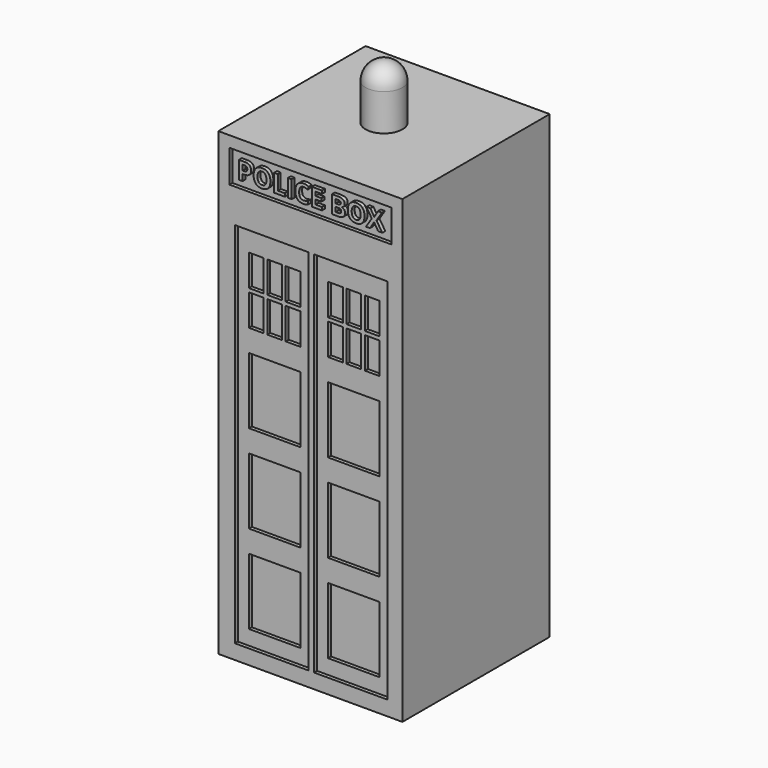
from build123d import *

# Parameters (mm, degrees)
F0_W      = 50
F0_H      = 50
F1_DEPTH  = 125
F6_W      = 44
F6_H      = 8.8186975504
F6_W_2    = 1.0133068417
F6_H_2    = 4.7779143029
F7_DEPTH  = 1
F6_W_3    = 4
F6_H_3    = 8.5
F6_W_4    = 14
F6_H_4    = 18
F8_DEPTH  = 2
F6_W_5    = 20
F6_H_5    = 100
F9_DEPTH  = 1
F11_W     = 44
F11_H     = 22
F11_W_2   = 1.2572977775
F11_H_2   = 4.6096520825
F11_H_3   = 6.4157807891
F12_DEPTH = 1


with BuildPart() as f1:
    # F0 (on Top) → F1 (new body)
    with BuildSketch(Plane.XY):
        Rectangle(F0_W, F0_H)
    extrude(amount=F1_DEPTH)

    # F3 (on Front) → F4 (revolve)
    with BuildSketch(Plane.XZ):
        with BuildLine():
            Line((0, 125), (0, 140))
            ThreePointArc((0, 140), (-3.5355339059, 138.5355339059), (-5, 135))
            Line((-5, 135), (-5, 125))
            Line((-5, 125), (0, 125))
        make_face()
    revolve(axis=Axis((0, 0, 66.3798125461), (0, 0, 1)))

    # F6 (on offset) → F7 (cut)
    with BuildSketch(Plane.XZ.offset(25)):
        with Locations((0, 117.5906512248)):
            Rectangle(F6_W, F6_H)
        with BuildLine():
            add(Edge.make_bspline(
                [(-16.5506784136, 119.584847455), (-16.0984026561, 119.2104781574), (-16.0984026561, 118.4690596324)],
                knots=[0, 0, 0, 1, 1, 1], degree=2))
            add(Edge.make_bspline(
                [(-16.0984026561, 118.4690596324), (-16.0984026561, 117.6973151029), (-16.580481556, 117.2889597658)],
                knots=[0, 0, 0, 1, 1, 1], degree=2))
            add(Edge.make_bspline(
                [(-16.580481556, 117.2889597658), (-17.0625604559, 116.8806044286), (-17.9514261065, 116.8806044286)],
                knots=[0, 0, 0, 1, 1, 1], degree=2))
            Line((-17.9514261065, 116.8806044286), (-18.3854016888, 116.8806044286))
            Line((-18.3854016888, 116.8806044286), (-18.3854016888, 115.1813024496))
            Line((-18.3854016888, 115.1813024496), (-19.3987085305, 115.1813024496))
            Line((-19.3987085305, 115.1813024496), (-19.3987085305, 119.9592167525))
            Line((-19.3987085305, 119.9592167525), (-17.8729967844, 119.9592167525))
            add(Edge.make_bspline(
                [(-17.8729967844, 119.9592167525), (-17.0029541711, 119.9592167525), (-16.5506784136, 119.584847455)],
                knots=[0, 0, 0, 1, 1, 1], degree=2))
        make_face(mode=Mode.SUBTRACT)
        with BuildLine():
            add(Edge.make_bspline(
                [(-11.4428380957, 119.4002771169), (-10.8593239392, 118.7660453321), (-10.8593239392, 117.577056809)],
                knots=[0, 0, 0, 1, 1, 1], degree=2))
            add(Edge.make_bspline(
                [(-10.8593239392, 117.577056809), (-10.8593239392, 116.3901597344), (-11.4475438551, 115.7527907767)],
                knots=[0, 0, 0, 1, 1, 1], degree=2))
            add(Edge.make_bspline(
                [(-11.4475438551, 115.7527907767), (-12.0357637709, 115.115421819), (-13.1337742804, 115.115421819)],
                knots=[0, 0, 0, 1, 1, 1], degree=2))
            add(Edge.make_bspline(
                [(-13.1337742804, 115.115421819), (-14.2317847899, 115.115421819), (-14.8200047058, 115.7527907767)],
                knots=[0, 0, 0, 1, 1, 1], degree=2))
            add(Edge.make_bspline(
                [(-14.8200047058, 115.7527907767), (-15.4082246216, 116.3901597344), (-15.4082246216, 117.5833311547)],
                knots=[0, 0, 0, 1, 1, 1], degree=2))
            add(Edge.make_bspline(
                [(-15.4082246216, 117.5833311547), (-15.4082246216, 118.7765025751), (-14.8184361193, 119.4055057384)],
                knots=[0, 0, 0, 1, 1, 1], degree=2))
            add(Edge.make_bspline(
                [(-14.8184361193, 119.4055057384), (-14.2286476171, 120.0345089017), (-13.1274999346, 120.0345089017)],
                knots=[0, 0, 0, 1, 1, 1], degree=2))
            add(Edge.make_bspline(
                [(-13.1274999346, 120.0345089017), (-12.0263522522, 120.0345089017), (-11.4428380957, 119.4002771169)],
                knots=[0, 0, 0, 1, 1, 1], degree=2))
        make_face(mode=Mode.SUBTRACT)
        Polygon((-6.9179890722, 115.1813024496), (-9.8690230321, 115.1813024496), (-9.8690230321, 119.9592167525), (-8.8557161904, 119.9592167525), (-8.8557161904, 116.0178818854), (-6.9179890722, 116.0178818854), align=None, mode=Mode.SUBTRACT)
        with Locations((-5.5810305613, 117.5702596011)):
            Rectangle(F6_W_2, F6_H_2, mode=Mode.SUBTRACT)
        with BuildLine():
            add(Edge.make_bspline(
                [(-1.3097696792, 119.0896970014), (-1.5806122716, 119.1843350501), (-1.8420433453, 119.1843350501)],
                knots=[0, 0, 0, 1, 1, 1], degree=2))
            add(Edge.make_bspline(
                [(-1.8420433453, 119.1843350501), (-2.4140545345, 119.1843350501), (-2.727771823, 118.7545423649)],
                knots=[0, 0, 0, 1, 1, 1], degree=2))
            add(Edge.make_bspline(
                [(-2.727771823, 118.7545423649), (-3.0414891114, 118.3247496797), (-3.0414891114, 117.5571880474)],
                knots=[0, 0, 0, 1, 1, 1], degree=2))
            add(Edge.make_bspline(
                [(-3.0414891114, 117.5571880474), (-3.0414891114, 115.9593213249), (-1.8420433453, 115.9593213249)],
                knots=[0, 0, 0, 1, 1, 1], degree=2))
            add(Edge.make_bspline(
                [(-1.8420433453, 115.9593213249), (-1.3390499595, 115.9593213249), (-0.6237745418, 116.2102951557)],
                knots=[0, 0, 0, 1, 1, 1], degree=2))
            Line((-0.6237745418, 116.2102951557), (-0.6237745418, 115.3611670283))
            add(Edge.make_bspline(
                [(-0.6237745418, 115.3611670283), (-1.2114715955, 115.115421819), (-1.9372042561, 115.115421819)],
                knots=[0, 0, 0, 1, 1, 1], degree=2))
            add(Edge.make_bspline(
                [(-1.9372042561, 115.115421819), (-2.979791378, 115.115421819), (-3.5319338057, 115.7480850174)],
                knots=[0, 0, 0, 1, 1, 1], degree=2))
            add(Edge.make_bspline(
                [(-3.5319338057, 115.7480850174), (-4.0840762333, 116.3807482157), (-4.0840762333, 117.5634623931)],
                knots=[0, 0, 0, 1, 1, 1], degree=2))
            add(Edge.make_bspline(
                [(-4.0840762333, 117.5634623931), (-4.0840762333, 118.3090638153), (-3.8127107788, 118.8695720373)],
                knots=[0, 0, 0, 1, 1, 1], degree=2))
            add(Edge.make_bspline(
                [(-3.8127107788, 118.8695720373), (-3.5413453243, 119.4300802593), (-3.033123317, 119.7286345455)],
                knots=[0, 0, 0, 1, 1, 1], degree=2))
            add(Edge.make_bspline(
                [(-3.033123317, 119.7286345455), (-2.5249013098, 120.0271888317), (-1.8420433453, 120.0271888317)],
                knots=[0, 0, 0, 1, 1, 1], degree=2))
            add(Edge.make_bspline(
                [(-1.8420433453, 120.0271888317), (-1.1466366892, 120.0271888317), (-0.4439099631, 119.691511333)],
                knots=[0, 0, 0, 1, 1, 1], degree=2))
            Line((-0.4439099631, 119.691511333), (-0.7701759431, 118.8674805887))
            add(Edge.make_bspline(
                [(-0.7701759431, 118.8674805887), (-1.0389270869, 118.9950589527), (-1.3097696792, 119.0896970014)],
                knots=[0, 0, 0, 1, 1, 1], degree=2))
        make_face(mode=Mode.SUBTRACT)
        Polygon((3.1439700923, 116.0178818854), (3.1439700923, 115.1813024496), (0.3926694727, 115.1813024496), (0.3926694727, 119.9592167525), (3.1439700923, 119.9592167525), (3.1439700923, 119.1289116624), (1.4059763143, 119.1289116624), (1.4059763143, 118.0800501948), (3.0237117984, 118.0800501948), (3.0237117984, 117.2497451047), (1.4059763143, 117.2497451047), (1.4059763143, 116.0178818854), align=None, mode=Mode.SUBTRACT)
        with BuildLine():
            Line((5.8795848475, 115.1813024496), (5.8795848475, 119.9592167525))
            Line((5.8795848475, 119.9592167525), (7.3666047946, 119.9592167525))
            add(Edge.make_bspline(
                [(7.3666047946, 119.9592167525), (8.3830488092, 119.9592167525), (8.8421217746, 119.670073985)],
                knots=[0, 0, 0, 1, 1, 1], degree=2))
            add(Edge.make_bspline(
                [(8.8421217746, 119.670073985), (9.30119474, 119.3809312175), (9.30119474, 118.7503594677)],
                knots=[0, 0, 0, 1, 1, 1], degree=2))
            add(Edge.make_bspline(
                [(9.30119474, 118.7503594677), (9.30119474, 118.3216125069), (9.1004156754, 118.0471098795)],
                knots=[0, 0, 0, 1, 1, 1], degree=2))
            add(Edge.make_bspline(
                [(9.1004156754, 118.0471098795), (8.8996366108, 117.7726072521), (8.5660505608, 117.7171838645)],
                knots=[0, 0, 0, 1, 1, 1], degree=2))
            Line((8.5660505608, 117.7171838645), (8.5660505608, 117.6847664113))
            add(Edge.make_bspline(
                [(8.5660505608, 117.6847664113), (9.0198949047, 117.5833311547), (9.2211968315, 117.3056913545)],
                knots=[0, 0, 0, 1, 1, 1], degree=2))
            add(Edge.make_bspline(
                [(9.2211968315, 117.3056913545), (9.4224987582, 117.0280515542), (9.4224987582, 116.5668871402)],
                knots=[0, 0, 0, 1, 1, 1], degree=2))
            add(Edge.make_bspline(
                [(9.4224987582, 116.5668871402), (9.4224987582, 115.913309456), (8.949831377, 115.5473059528)],
                knots=[0, 0, 0, 1, 1, 1], degree=2))
            add(Edge.make_bspline(
                [(8.949831377, 115.5473059528), (8.4771639957, 115.1813024496), (7.6667276673, 115.1813024496)],
                knots=[0, 0, 0, 1, 1, 1], degree=2))
            Line((7.6667276673, 115.1813024496), (5.8795848475, 115.1813024496))
        make_face(mode=Mode.SUBTRACT)
        with BuildLine():
            add(Edge.make_bspline(
                [(14.1293038091, 119.4002771169), (14.7128179655, 118.7660453321), (14.7128179655, 117.577056809)],
                knots=[0, 0, 0, 1, 1, 1], degree=2))
            add(Edge.make_bspline(
                [(14.7128179655, 117.577056809), (14.7128179655, 116.3901597344), (14.1245980497, 115.7527907767)],
                knots=[0, 0, 0, 1, 1, 1], degree=2))
            add(Edge.make_bspline(
                [(14.1245980497, 115.7527907767), (13.5363781339, 115.115421819), (12.4383676244, 115.115421819)],
                knots=[0, 0, 0, 1, 1, 1], degree=2))
            add(Edge.make_bspline(
                [(12.4383676244, 115.115421819), (11.3403571148, 115.115421819), (10.752137199, 115.7527907767)],
                knots=[0, 0, 0, 1, 1, 1], degree=2))
            add(Edge.make_bspline(
                [(10.752137199, 115.7527907767), (10.1639172832, 116.3901597344), (10.1639172832, 117.5833311547)],
                knots=[0, 0, 0, 1, 1, 1], degree=2))
            add(Edge.make_bspline(
                [(10.1639172832, 117.5833311547), (10.1639172832, 118.7765025751), (10.7537057855, 119.4055057384)],
                knots=[0, 0, 0, 1, 1, 1], degree=2))
            add(Edge.make_bspline(
                [(10.7537057855, 119.4055057384), (11.3434942877, 120.0345089017), (12.4446419701, 120.0345089017)],
                knots=[0, 0, 0, 1, 1, 1], degree=2))
            add(Edge.make_bspline(
                [(12.4446419701, 120.0345089017), (13.5457896526, 120.0345089017), (14.1293038091, 119.4002771169)],
                knots=[0, 0, 0, 1, 1, 1], degree=2))
        make_face(mode=Mode.SUBTRACT)
        Polygon((17.9514261065, 117.5896055005), (19.5660244177, 115.1813024496), (18.4094533476, 115.1813024496), (17.2978484223, 116.988314031), (16.1872892212, 115.1813024496), (15.1018274032, 115.1813024496), (16.6871454341, 117.6450288881), (15.2032626598, 119.9592167525), (16.3211419309, 119.9592167525), (17.350134637, 118.2400460119), (18.3603043058, 119.9592167525), (19.4509947452, 119.9592167525), align=None, mode=Mode.SUBTRACT)
        with BuildLine():
            add(Edge.make_bspline(
                [(-14.0388486576, 118.7838226452), (-14.3457687381, 118.3770358945), (-14.3457687381, 117.577056809)],
                knots=[0, 0, 0, 1, 1, 1], degree=2))
            add(Edge.make_bspline(
                [(-14.3457687381, 117.577056809), (-14.3457687381, 116.7760319992), (-14.0419858304, 116.3708138349)],
                knots=[0, 0, 0, 1, 1, 1], degree=2))
            add(Edge.make_bspline(
                [(-14.0419858304, 116.3708138349), (-13.7382029228, 115.9655956707), (-13.1337742804, 115.9655956707)],
                knots=[0, 0, 0, 1, 1, 1], degree=2))
            add(Edge.make_bspline(
                [(-13.1337742804, 115.9655956707), (-11.9217798227, 115.9655956707), (-11.9217798227, 117.577056809)],
                knots=[0, 0, 0, 1, 1, 1], degree=2))
            add(Edge.make_bspline(
                [(-11.9217798227, 117.577056809), (-11.9217798227, 119.1906093958), (-13.1274999346, 119.1906093958)],
                knots=[0, 0, 0, 1, 1, 1], degree=2))
            add(Edge.make_bspline(
                [(-13.1274999346, 119.1906093958), (-13.731928577, 119.1906093958), (-14.0388486576, 118.7838226452)],
                knots=[0, 0, 0, 1, 1, 1], degree=2))
        make_face()
        with BuildLine():
            Line((-18.3854016888, 119.1289116624), (-18.3854016888, 117.7109095187))
            Line((-18.3854016888, 117.7109095187), (-18.0518156388, 117.7109095187))
            add(Edge.make_bspline(
                [(-18.0518156388, 117.7109095187), (-17.5854226033, 117.7109095187), (-17.3532718099, 117.8954798567)],
                knots=[0, 0, 0, 1, 1, 1], degree=2))
            add(Edge.make_bspline(
                [(-17.3532718099, 117.8954798567), (-17.1211210164, 118.0800501948), (-17.1211210164, 118.4324592821)],
                knots=[0, 0, 0, 1, 1, 1], degree=2))
            add(Edge.make_bspline(
                [(-17.1211210164, 118.4324592821), (-17.1211210164, 118.7890512666), (-17.3156257353, 118.9589814645)],
                knots=[0, 0, 0, 1, 1, 1], degree=2))
            add(Edge.make_bspline(
                [(-17.3156257353, 118.9589814645), (-17.5101304541, 119.1289116624), (-17.9252829991, 119.1289116624)],
                knots=[0, 0, 0, 1, 1, 1], degree=2))
            Line((-17.9252829991, 119.1289116624), (-18.3854016888, 119.1289116624))
        make_face()
        with BuildLine():
            add(Edge.make_bspline(
                [(11.5332932472, 118.7838226452), (11.2263731667, 118.3770358945), (11.2263731667, 117.577056809)],
                knots=[0, 0, 0, 1, 1, 1], degree=2))
            add(Edge.make_bspline(
                [(11.2263731667, 117.577056809), (11.2263731667, 116.7760319992), (11.5301560744, 116.3708138349)],
                knots=[0, 0, 0, 1, 1, 1], degree=2))
            add(Edge.make_bspline(
                [(11.5301560744, 116.3708138349), (11.833938982, 115.9655956707), (12.4383676244, 115.9655956707)],
                knots=[0, 0, 0, 1, 1, 1], degree=2))
            add(Edge.make_bspline(
                [(12.4383676244, 115.9655956707), (13.650362082, 115.9655956707), (13.650362082, 117.577056809)],
                knots=[0, 0, 0, 1, 1, 1], degree=2))
            add(Edge.make_bspline(
                [(13.650362082, 117.577056809), (13.650362082, 119.1906093958), (12.4446419701, 119.1906093958)],
                knots=[0, 0, 0, 1, 1, 1], degree=2))
            add(Edge.make_bspline(
                [(12.4446419701, 119.1906093958), (11.8402133278, 119.1906093958), (11.5332932472, 118.7838226452)],
                knots=[0, 0, 0, 1, 1, 1], degree=2))
        make_face()
        with BuildLine():
            Line((6.8928916891, 119.1289116624), (6.8928916891, 118.0664557789))
            Line((6.8928916891, 118.0664557789), (7.4805887428, 118.0664557789))
            add(Edge.make_bspline(
                [(7.4805887428, 118.0664557789), (7.8926041149, 118.0664557789), (8.077174453, 118.1940341429)],
                knots=[0, 0, 0, 1, 1, 1], degree=2))
            add(Edge.make_bspline(
                [(8.077174453, 118.1940341429), (8.261744791, 118.3216125069), (8.261744791, 118.6154610337)],
                knots=[0, 0, 0, 1, 1, 1], degree=2))
            add(Edge.make_bspline(
                [(8.261744791, 118.6154610337), (8.261744791, 118.8904865232), (8.0609657264, 119.0096990928)],
                knots=[0, 0, 0, 1, 1, 1], degree=2))
            add(Edge.make_bspline(
                [(8.0609657264, 119.0096990928), (7.8601866618, 119.1289116624), (7.4251653552, 119.1289116624)],
                knots=[0, 0, 0, 1, 1, 1], degree=2))
            Line((7.4251653552, 119.1289116624), (6.8928916891, 119.1289116624))
        make_face()
        with BuildLine():
            Line((7.520326266, 117.2633395205), (6.8928916891, 117.2633395205))
            Line((6.8928916891, 117.2633395205), (6.8928916891, 116.0178818854))
            Line((6.8928916891, 116.0178818854), (7.5527437191, 116.0178818854))
            add(Edge.make_bspline(
                [(7.5527437191, 116.0178818854), (7.971033437, 116.0178818854), (8.1702439152, 116.1778777025)],
                knots=[0, 0, 0, 1, 1, 1], degree=2))
            add(Edge.make_bspline(
                [(8.1702439152, 116.1778777025), (8.3694543933, 116.3378735196), (8.3694543933, 116.6683223968)],
                knots=[0, 0, 0, 1, 1, 1], degree=2))
            add(Edge.make_bspline(
                [(8.3694543933, 116.6683223968), (8.3694543933, 117.2633395205), (7.520326266, 117.2633395205)],
                knots=[0, 0, 0, 1, 1, 1], degree=2))
        make_face()
    extrude(amount=-F7_DEPTH, mode=Mode.SUBTRACT)

    # F6 (on offset) → F8 (cut)
    with BuildSketch(Plane.XZ.offset(25)):
        with Locations((-15.5, 93.75)):
            Rectangle(F6_W_3, F6_H_3)
        with Locations((-10.5, 93.75)):
            Rectangle(F6_W_3, F6_H_3)
        with Locations((-5.5, 93.75)):
            Rectangle(F6_W_3, F6_H_3)
        with Locations((6, 93.75)):
            Rectangle(F6_W_3, F6_H_3)
        with Locations((11, 93.75)):
            Rectangle(F6_W_3, F6_H_3)
        with Locations((16, 93.75)):
            Rectangle(F6_W_3, F6_H_3)
        with Locations((16, 84.25)):
            Rectangle(F6_W_3, F6_H_3)
        with Locations((11, 84.25)):
            Rectangle(F6_W_3, F6_H_3)
        with Locations((6, 84.25)):
            Rectangle(F6_W_3, F6_H_3)
        with Locations((-5.5, 84.25)):
            Rectangle(F6_W_3, F6_H_3)
        with Locations((-10.5, 84.25)):
            Rectangle(F6_W_3, F6_H_3)
        with Locations((-15.5, 84.25)):
            Rectangle(F6_W_3, F6_H_3)
        with Locations((-10.5, 65)):
            Rectangle(F6_W_4, F6_H_4)
        with Locations((11, 65)):
            Rectangle(F6_W_4, F6_H_4)
        with Locations((-10.5, 41)):
            Rectangle(F6_W_4, F6_H_4)
        with Locations((11, 41)):
            Rectangle(F6_W_4, F6_H_4)
        with Locations((-10.5, 17)):
            Rectangle(F6_W_4, F6_H_4)
        with Locations((11, 17)):
            Rectangle(F6_W_4, F6_H_4)
    extrude(amount=-F8_DEPTH, mode=Mode.SUBTRACT)

    # F6 (on offset) → F9 (cut)
    with BuildSketch(Plane.XZ.offset(25)):
        with Locations((-10.5, 54)):
            Rectangle(F6_W_5, F6_H_5)
        with Locations((-10.5, 17)):
            Rectangle(F6_W_4, F6_H_4, mode=Mode.SUBTRACT)
        with Locations((-10.5, 41)):
            Rectangle(F6_W_4, F6_H_4, mode=Mode.SUBTRACT)
        with Locations((-10.5, 65)):
            Rectangle(F6_W_4, F6_H_4, mode=Mode.SUBTRACT)
        Polygon((-17.5, 89.5), (-17.5, 98), (-13.5, 98), (-12.5, 98), (-8.5, 98), (-7.5, 98), (-3.5, 98), (-3.5, 89.5), (-3.5, 88.5), (-3.5, 80), (-7.5, 80), (-8.5, 80), (-12.5, 80), (-13.5, 80), (-17.5, 80), (-17.5, 88.5), align=None, mode=Mode.SUBTRACT)
        with Locations((11, 54)):
            Rectangle(F6_W_5, F6_H_5)
        with Locations((11, 17)):
            Rectangle(F6_W_4, F6_H_4, mode=Mode.SUBTRACT)
        with Locations((11, 41)):
            Rectangle(F6_W_4, F6_H_4, mode=Mode.SUBTRACT)
        with Locations((11, 65)):
            Rectangle(F6_W_4, F6_H_4, mode=Mode.SUBTRACT)
        Polygon((4, 89.5), (4, 98), (8, 98), (9, 98), (13, 98), (14, 98), (18, 98), (18, 89.5), (18, 88.5), (18, 80), (14, 80), (13, 80), (9, 80), (8, 80), (4, 80), (4, 88.5), align=None, mode=Mode.SUBTRACT)
        Polygon((-12.5, 98), (-13.5, 98), (-13.5, 89.5), (-17.5, 89.5), (-17.5, 88.5), (-13.5, 88.5), (-13.5, 80), (-12.5, 80), (-12.5, 88.5), (-8.5, 88.5), (-8.5, 80), (-7.5, 80), (-7.5, 88.5), (-3.5, 88.5), (-3.5, 89.5), (-7.5, 89.5), (-7.5, 98), (-8.5, 98), (-8.5, 89.5), (-12.5, 89.5), align=None)
        Polygon((9, 98), (8, 98), (8, 89.5), (4, 89.5), (4, 88.5), (8, 88.5), (8, 80), (9, 80), (9, 88.5), (13, 88.5), (13, 80), (14, 80), (14, 88.5), (18, 88.5), (18, 89.5), (14, 89.5), (14, 98), (13, 98), (13, 89.5), (9, 89.5), align=None)
    extrude(amount=-F9_DEPTH, mode=Mode.SUBTRACT)

    # F11 (on offset) → F12 (cut)
    with BuildSketch(Plane(origin=(0, 25, 0), x_dir=(-1, 0, 0), z_dir=(0, 1, 0))):
        with Locations((0, 94)):
            Rectangle(F11_W, F11_H)
        with BuildLine():
            Line((-12.5178772498, 87.1539132077), (-12.5178772498, 88.218592438))
            Line((-12.5178772498, 88.218592438), (-10.1259770708, 88.218592438))
            Line((-10.1259770708, 88.218592438), (-10.1259770708, 85.0931586133))
            add(Edge.make_bspline(
                [(-10.1259770708, 85.0931586133), (-10.7077906278, 84.9031786763), (-11.2210003187, 84.8266589795)],
                knots=[0, 0, 0, 1, 1, 1], degree=2))
            add(Edge.make_bspline(
                [(-11.2210003187, 84.8266589795), (-11.7342100097, 84.7501392826), (-12.2698478876, 84.7501392826)],
                knots=[0, 0, 0, 1, 1, 1], degree=2))
            add(Edge.make_bspline(
                [(-12.2698478876, 84.7501392826), (-13.6340093796, 84.7501392826), (-14.3536903215, 85.5522767944)],
                knots=[0, 0, 0, 1, 1, 1], degree=2))
            add(Edge.make_bspline(
                [(-14.3536903215, 85.5522767944), (-15.0733712634, 86.3544143062), (-15.0733712634, 87.8557835305)],
                knots=[0, 0, 0, 1, 1, 1], degree=2))
            add(Edge.make_bspline(
                [(-15.0733712634, 87.8557835305), (-15.0733712634, 89.3149349911), (-14.2382511237, 90.1309252066)],
                knots=[0, 0, 0, 1, 1, 1], degree=2))
            add(Edge.make_bspline(
                [(-14.2382511237, 90.1309252066), (-13.403130984, 90.9469154221), (-11.9241899467, 90.9469154221)],
                knots=[0, 0, 0, 1, 1, 1], degree=2))
            add(Edge.make_bspline(
                [(-11.9241899467, 90.9469154221), (-10.9953991436, 90.9469154221), (-10.1338929015, 90.5761906839)],
                knots=[0, 0, 0, 1, 1, 1], degree=2))
            Line((-10.1338929015, 90.5761906839), (-10.5587091495, 89.5537292175))
            add(Edge.make_bspline(
                [(-10.5587091495, 89.5537292175), (-11.2183617085, 89.883555497), (-11.9321057774, 89.883555497)],
                knots=[0, 0, 0, 1, 1, 1], degree=2))
            add(Edge.make_bspline(
                [(-11.9321057774, 89.883555497), (-12.7606293915, 89.883555497), (-13.2593267261, 89.3268087372)],
                knots=[0, 0, 0, 1, 1, 1], degree=2))
            add(Edge.make_bspline(
                [(-13.2593267261, 89.3268087372), (-13.7580240607, 88.7700619773), (-13.7580240607, 87.8307167333)],
                knots=[0, 0, 0, 1, 1, 1], degree=2))
            add(Edge.make_bspline(
                [(-13.7580240607, 87.8307167333), (-13.7580240607, 86.8491537255), (-13.3562956523, 86.3319861192)],
                knots=[0, 0, 0, 1, 1, 1], degree=2))
            add(Edge.make_bspline(
                [(-13.3562956523, 86.3319861192), (-12.9545672439, 85.8148185129), (-12.1880509703, 85.8148185129)],
                knots=[0, 0, 0, 1, 1, 1], degree=2))
            add(Edge.make_bspline(
                [(-12.1880509703, 85.8148185129), (-11.7869822144, 85.8148185129), (-11.3753590175, 85.8966154302)],
                knots=[0, 0, 0, 1, 1, 1], degree=2))
            Line((-11.3753590175, 85.8966154302), (-11.3753590175, 87.1539132077))
            Line((-11.3753590175, 87.1539132077), (-12.5178772498, 87.1539132077))
        make_face(mode=Mode.SUBTRACT)
        with BuildLine():
            Line((-4.5611480828, 84.8332555051), (-5.5255601241, 84.8332555051))
            Line((-5.5255601241, 84.8332555051), (-5.6944311792, 85.4229848928))
            Line((-5.6944311792, 85.4229848928), (-5.7603964351, 85.4229848928))
            add(Edge.make_bspline(
                [(-5.7603964351, 85.4229848928), (-5.9622501182, 85.101074444), (-6.3336345089, 84.9256068633)],
                knots=[0, 0, 0, 1, 1, 1], degree=2))
            add(Edge.make_bspline(
                [(-6.3336345089, 84.9256068633), (-6.7050188997, 84.7501392826), (-7.178649437, 84.7501392826)],
                knots=[0, 0, 0, 1, 1, 1], degree=2))
            add(Edge.make_bspline(
                [(-7.178649437, 84.7501392826), (-7.9913413898, 84.7501392826), (-8.4036242391, 85.1855099716)],
                knots=[0, 0, 0, 1, 1, 1], degree=2))
            add(Edge.make_bspline(
                [(-8.4036242391, 85.1855099716), (-8.8159070885, 85.6208806606), (-8.8159070885, 86.4375305286)],
                knots=[0, 0, 0, 1, 1, 1], degree=2))
            Line((-8.8159070885, 86.4375305286), (-8.8159070885, 89.4429075875))
            Line((-8.8159070885, 89.4429075875), (-7.558609311, 89.4429075875))
            Line((-7.558609311, 89.4429075875), (-7.558609311, 86.7502058416))
            add(Edge.make_bspline(
                [(-7.558609311, 86.7502058416), (-7.558609311, 86.251508507), (-7.3811627727, 86.0021598397)],
                knots=[0, 0, 0, 1, 1, 1], degree=2))
            add(Edge.make_bspline(
                [(-7.3811627727, 86.0021598397), (-7.2037162343, 85.7528111724), (-6.8158405296, 85.7528111724)],
                knots=[0, 0, 0, 1, 1, 1], degree=2))
            add(Edge.make_bspline(
                [(-6.8158405296, 85.7528111724), (-6.2881184824, 85.7528111724), (-6.0532821713, 86.1050656389)],
                knots=[0, 0, 0, 1, 1, 1], degree=2))
            add(Edge.make_bspline(
                [(-6.0532821713, 86.1050656389), (-5.8184458603, 86.4573201054), (-5.8184458603, 87.2739699735)],
                knots=[0, 0, 0, 1, 1, 1], degree=2))
            Line((-5.8184458603, 87.2739699735), (-5.8184458603, 89.4429075875))
            Line((-5.8184458603, 89.4429075875), (-4.5611480828, 89.4429075875))
            Line((-4.5611480828, 89.4429075875), (-4.5611480828, 84.8332555051))
        make_face(mode=Mode.SUBTRACT)
        with Locations((-2.613194076, 87.1380815463)):
            Rectangle(F11_W_2, F11_H_2, mode=Mode.SUBTRACT)
        with Locations((-0.0365911805, 88.0411458996)):
            Rectangle(F11_W_2, F11_H_3, mode=Mode.SUBTRACT)
        with BuildLine():
            add(Edge.make_bspline(
                [(-2.6112151184, 90.0154860088), (-3.2959344746, 90.0154860088), (-3.2959344746, 90.6342401091)],
                knots=[0, 0, 0, 1, 1, 1], degree=2))
            add(Edge.make_bspline(
                [(-3.2959344746, 90.6342401091), (-3.2959344746, 91.2490362941), (-2.6112151184, 91.2490362941)],
                knots=[0, 0, 0, 1, 1, 1], degree=2))
            add(Edge.make_bspline(
                [(-2.6112151184, 91.2490362941), (-1.9264957621, 91.2490362941), (-1.9264957621, 90.6342401091)],
                knots=[0, 0, 0, 1, 1, 1], degree=2))
            add(Edge.make_bspline(
                [(-1.9264957621, 90.6342401091), (-1.9264957621, 90.3413543729), (-2.0973457749, 90.1784201909)],
                knots=[0, 0, 0, 1, 1, 1], degree=2))
            add(Edge.make_bspline(
                [(-2.0973457749, 90.1784201909), (-2.2681957877, 90.0154860088), (-2.6112151184, 90.0154860088)],
                knots=[0, 0, 0, 1, 1, 1], degree=2))
        make_face(mode=Mode.SUBTRACT)
        with Locations((2.5400117151, 88.0411458996)):
            Rectangle(F11_W_2, F11_H_3, mode=Mode.SUBTRACT)
        with Locations((5.1166146106, 87.1380815463)):
            Rectangle(F11_W_2, F11_H_2, mode=Mode.SUBTRACT)
        with BuildLine():
            Line((11.3193276231, 87.838632564), (11.3193276231, 84.8332555051))
            Line((11.3193276231, 84.8332555051), (10.0620298456, 84.8332555051))
            Line((10.0620298456, 84.8332555051), (10.0620298456, 87.525957251))
            add(Edge.make_bspline(
                [(10.0620298456, 87.525957251), (10.0620298456, 88.0246545856), (9.8845833072, 88.2740032529)],
                knots=[0, 0, 0, 1, 1, 1], degree=2))
            add(Edge.make_bspline(
                [(9.8845833072, 88.2740032529), (9.7071367689, 88.5233519203), (9.3192610642, 88.5233519203)],
                knots=[0, 0, 0, 1, 1, 1], degree=2))
            add(Edge.make_bspline(
                [(9.3192610642, 88.5233519203), (8.7915390169, 88.5233519203), (8.5567027059, 88.1710974537)],
                knots=[0, 0, 0, 1, 1, 1], degree=2))
            add(Edge.make_bspline(
                [(8.5567027059, 88.1710974537), (8.3218663949, 87.8188429872), (8.3218663949, 87.0021931192)],
                knots=[0, 0, 0, 1, 1, 1], degree=2))
            Line((8.3218663949, 87.0021931192), (8.3218663949, 84.8332555051))
            Line((8.3218663949, 84.8332555051), (7.0645686174, 84.8332555051))
            Line((7.0645686174, 84.8332555051), (7.0645686174, 89.4429075875))
            Line((7.0645686174, 89.4429075875), (8.0250227434, 89.4429075875))
            Line((8.0250227434, 89.4429075875), (8.1938937985, 88.8531781998))
            Line((8.1938937985, 88.8531781998), (8.2638169697, 88.8531781998))
            add(Edge.make_bspline(
                [(8.2638169697, 88.8531781998), (8.4749057886, 89.1869623946), (8.8436515691, 89.3578124074)],
                knots=[0, 0, 0, 1, 1, 1], degree=2))
            add(Edge.make_bspline(
                [(8.8436515691, 89.3578124074), (9.2123973496, 89.5286624202), (9.6820699716, 89.5286624202)],
                knots=[0, 0, 0, 1, 1, 1], degree=2))
            add(Edge.make_bspline(
                [(9.6820699716, 89.5286624202), (10.4868460936, 89.5286624202), (10.9030868584, 89.0939513838)],
                knots=[0, 0, 0, 1, 1, 1], degree=2))
            add(Edge.make_bspline(
                [(10.9030868584, 89.0939513838), (11.3193276231, 88.6592403474), (11.3193276231, 87.838632564)],
                knots=[0, 0, 0, 1, 1, 1], degree=2))
        make_face(mode=Mode.SUBTRACT)
        with BuildLine():
            add(Edge.make_bspline(
                [(15.6149850875, 84.8306168948), (15.240302434, 84.7501392826), (14.6993873356, 84.7501392826)],
                knots=[0, 0, 0, 1, 1, 1], degree=2))
            add(Edge.make_bspline(
                [(14.6993873356, 84.7501392826), (13.587213121, 84.7501392826), (12.96054319, 85.3649354677)],
                knots=[0, 0, 0, 1, 1, 1], degree=2))
            add(Edge.make_bspline(
                [(12.96054319, 85.3649354677), (12.3338732589, 85.9797316527), (12.3338732589, 87.1050989184)],
                knots=[0, 0, 0, 1, 1, 1], degree=2))
            add(Edge.make_bspline(
                [(12.3338732589, 87.1050989184), (12.3338732589, 88.263448812), (12.9130482057, 88.8960556161)],
                knots=[0, 0, 0, 1, 1, 1], degree=2))
            add(Edge.make_bspline(
                [(12.9130482057, 88.8960556161), (13.4922231526, 89.5286624202), (14.514684619, 89.5286624202)],
                knots=[0, 0, 0, 1, 1, 1], degree=2))
            add(Edge.make_bspline(
                [(14.514684619, 89.5286624202), (15.4909704064, 89.5286624202), (16.0351837676, 88.972575313)],
                knots=[0, 0, 0, 1, 1, 1], degree=2))
            add(Edge.make_bspline(
                [(16.0351837676, 88.972575313), (16.5793971288, 88.4164882057), (16.5793971288, 87.4349251979)],
                knots=[0, 0, 0, 1, 1, 1], degree=2))
            Line((16.5793971288, 87.4349251979), (16.5793971288, 86.8240869282))
            Line((16.5793971288, 86.8240869282), (13.6070026978, 86.8240869282))
            add(Edge.make_bspline(
                [(13.6070026978, 86.8240869282), (13.6281115797, 86.2884490503), (13.9249552313, 85.9876474834)],
                knots=[0, 0, 0, 1, 1, 1], degree=2))
            add(Edge.make_bspline(
                [(13.9249552313, 85.9876474834), (14.2217988828, 85.6868459165), (14.7574367608, 85.6868459165)],
                knots=[0, 0, 0, 1, 1, 1], degree=2))
            add(Edge.make_bspline(
                [(14.7574367608, 85.6868459165), (15.1743371781, 85.6868459165), (15.5450619162, 85.7732604017)],
                knots=[0, 0, 0, 1, 1, 1], degree=2))
            add(Edge.make_bspline(
                [(15.5450619162, 85.7732604017), (15.9157866544, 85.8596748869), (16.3194940205, 86.0496548239)],
                knots=[0, 0, 0, 1, 1, 1], degree=2))
            Line((16.3194940205, 86.0496548239), (16.3194940205, 85.0760076468))
            add(Edge.make_bspline(
                [(16.3194940205, 85.0760076468), (15.989667741, 84.911094507), (15.6149850875, 84.8306168948)],
                knots=[0, 0, 0, 1, 1, 1], degree=2))
        make_face(mode=Mode.SUBTRACT)
        with BuildLine():
            add(Edge.make_bspline(
                [(5.1185935683, 90.0154860088), (4.433874212, 90.0154860088), (4.433874212, 90.6342401091)],
                knots=[0, 0, 0, 1, 1, 1], degree=2))
            add(Edge.make_bspline(
                [(4.433874212, 90.6342401091), (4.433874212, 91.2490362941), (5.1185935683, 91.2490362941)],
                knots=[0, 0, 0, 1, 1, 1], degree=2))
            add(Edge.make_bspline(
                [(5.1185935683, 91.2490362941), (5.8033129246, 91.2490362941), (5.8033129246, 90.6342401091)],
                knots=[0, 0, 0, 1, 1, 1], degree=2))
            add(Edge.make_bspline(
                [(5.8033129246, 90.6342401091), (5.8033129246, 90.3413543729), (5.6324629118, 90.1784201909)],
                knots=[0, 0, 0, 1, 1, 1], degree=2))
            add(Edge.make_bspline(
                [(5.6324629118, 90.1784201909), (5.461612899, 90.0154860088), (5.1185935683, 90.0154860088)],
                knots=[0, 0, 0, 1, 1, 1], degree=2))
        make_face(mode=Mode.SUBTRACT)
        Polygon((-9.8660739625, 102.3443923369), (-9.8660739625, 96.3164872526), (-11.1405227065, 96.3164872526), (-11.1405227065, 98.9181569454), (-13.5271456651, 98.9181569454), (-13.5271456651, 96.3164872526), (-14.8055523245, 96.3164872526), (-14.8055523245, 102.3443923369), (-13.5271456651, 102.3443923369), (-13.5271456651, 99.9815168705), (-11.1405227065, 99.9815168705), (-11.1405227065, 102.3443923369), align=None, mode=Mode.SUBTRACT)
        with BuildLine():
            Line((-4.6389870848, 96.3164872526), (-5.5163249883, 96.3164872526))
            Line((-5.5163249883, 96.3164872526), (-5.7603964351, 96.9431571836))
            Line((-5.7603964351, 96.9431571836), (-5.7933790631, 96.9431571836))
            add(Edge.make_bspline(
                [(-5.7933790631, 96.9431571836), (-6.1100122914, 96.5434077329), (-6.4464350965, 96.3883893815)],
                knots=[0, 0, 0, 1, 1, 1], degree=2))
            add(Edge.make_bspline(
                [(-6.4464350965, 96.3883893815), (-6.7828579016, 96.2333710301), (-7.3224536949, 96.2333710301)],
                knots=[0, 0, 0, 1, 1, 1], degree=2))
            add(Edge.make_bspline(
                [(-7.3224536949, 96.2333710301), (-7.9860641693, 96.2333710301), (-8.3673433484, 96.6133309041)],
                knots=[0, 0, 0, 1, 1, 1], degree=2))
            add(Edge.make_bspline(
                [(-8.3673433484, 96.6133309041), (-8.7486225275, 96.9932907781), (-8.7486225275, 97.6938417958)],
                knots=[0, 0, 0, 1, 1, 1], degree=2))
            add(Edge.make_bspline(
                [(-8.7486225275, 97.6938417958), (-8.7486225275, 98.4273754415), (-8.2354128366, 98.7756719926)],
                knots=[0, 0, 0, 1, 1, 1], degree=2))
            add(Edge.make_bspline(
                [(-8.2354128366, 98.7756719926), (-7.7222031457, 99.1239685438), (-6.6878679331, 99.1609090871)],
                knots=[0, 0, 0, 1, 1, 1], degree=2))
            Line((-6.6878679331, 99.1609090871), (-5.8870497265, 99.1859758843))
            Line((-5.8870497265, 99.1859758843), (-5.8870497265, 99.3878295674))
            add(Edge.make_bspline(
                [(-5.8870497265, 99.3878295674), (-5.8870497265, 100.0883805851), (-6.6047517107, 100.0883805851)],
                knots=[0, 0, 0, 1, 1, 1], degree=2))
            add(Edge.make_bspline(
                [(-6.6047517107, 100.0883805851), (-7.1575405551, 100.0883805851), (-7.904267252, 99.7545963902)],
                knots=[0, 0, 0, 1, 1, 1], degree=2))
            Line((-7.904267252, 99.7545963902), (-8.3198483641, 100.6042288862))
            add(Edge.make_bspline(
                [(-8.3198483641, 100.6042288862), (-7.524307378, 101.0211293035), (-6.5559374213, 101.0211293035)],
                knots=[0, 0, 0, 1, 1, 1], degree=2))
            add(Edge.make_bspline(
                [(-6.5559374213, 101.0211293035), (-5.6284659233, 101.0211293035), (-5.1337265041, 100.6167622849)],
                knots=[0, 0, 0, 1, 1, 1], degree=2))
            add(Edge.make_bspline(
                [(-5.1337265041, 100.6167622849), (-4.6389870848, 100.2123952662), (-4.6389870848, 99.3878295674)],
                knots=[0, 0, 0, 1, 1, 1], degree=2))
            Line((-4.6389870848, 99.3878295674), (-4.6389870848, 96.3164872526))
        make_face(mode=Mode.SUBTRACT)
        with BuildLine():
            add(Edge.make_bspline(
                [(-1.5643465072, 100.775078899), (-1.199558642, 101.0118941677), (-0.7707844787, 101.0118941677)],
                knots=[0, 0, 0, 1, 1, 1], degree=2))
            add(Edge.make_bspline(
                [(-0.7707844787, 101.0118941677), (-0.5148392858, 101.0118941677), (-0.3459682307, 100.9749536244)],
                knots=[0, 0, 0, 1, 1, 1], degree=2))
            Line((-0.3459682307, 100.9749536244), (-0.4409581992, 99.796814154))
            add(Edge.make_bspline(
                [(-0.4409581992, 99.796814154), (-0.5939975929, 99.8377126126), (-0.8116829373, 99.8377126126)],
                knots=[0, 0, 0, 1, 1, 1], degree=2))
            add(Edge.make_bspline(
                [(-0.8116829373, 99.8377126126), (-1.4132860712, 99.8377126126), (-1.7497088763, 99.5283355625)],
                knots=[0, 0, 0, 1, 1, 1], degree=2))
            add(Edge.make_bspline(
                [(-1.7497088763, 99.5283355625), (-2.0861316814, 99.2189585123), (-2.0861316814, 98.6622117525)],
                knots=[0, 0, 0, 1, 1, 1], degree=2))
            Line((-2.0861316814, 98.6622117525), (-2.0861316814, 96.3164872526))
            Line((-2.0861316814, 96.3164872526), (-3.3434294589, 96.3164872526))
            Line((-3.3434294589, 96.3164872526), (-3.3434294589, 100.926139335))
            Line((-3.3434294589, 100.926139335), (-2.3908911636, 100.926139335))
            Line((-2.3908911636, 100.926139335), (-2.204869142, 100.1503879256))
            Line((-2.204869142, 100.1503879256), (-2.1441811066, 100.1503879256))
            add(Edge.make_bspline(
                [(-2.1441811066, 100.1503879256), (-1.9291343723, 100.5382636303), (-1.5643465072, 100.775078899)],
                knots=[0, 0, 0, 1, 1, 1], degree=2))
        make_face(mode=Mode.SUBTRACT)
        with BuildLine():
            add(Edge.make_bspline(
                [(2.2695541659, 100.775078899), (2.634342031, 101.0118941677), (3.0631161944, 101.0118941677)],
                knots=[0, 0, 0, 1, 1, 1], degree=2))
            add(Edge.make_bspline(
                [(3.0631161944, 101.0118941677), (3.3190613873, 101.0118941677), (3.4879324424, 100.9749536244)],
                knots=[0, 0, 0, 1, 1, 1], degree=2))
            Line((3.4879324424, 100.9749536244), (3.3929424739, 99.796814154))
            add(Edge.make_bspline(
                [(3.3929424739, 99.796814154), (3.2399030802, 99.8377126126), (3.0222177357, 99.8377126126)],
                knots=[0, 0, 0, 1, 1, 1], degree=2))
            add(Edge.make_bspline(
                [(3.0222177357, 99.8377126126), (2.4206146019, 99.8377126126), (2.0841917968, 99.5283355625)],
                knots=[0, 0, 0, 1, 1, 1], degree=2))
            add(Edge.make_bspline(
                [(2.0841917968, 99.5283355625), (1.7477689917, 99.2189585123), (1.7477689917, 98.6622117525)],
                knots=[0, 0, 0, 1, 1, 1], degree=2))
            Line((1.7477689917, 98.6622117525), (1.7477689917, 96.3164872526))
            Line((1.7477689917, 96.3164872526), (0.4904712142, 96.3164872526))
            Line((0.4904712142, 96.3164872526), (0.4904712142, 100.926139335))
            Line((0.4904712142, 100.926139335), (1.4430095094, 100.926139335))
            Line((1.4430095094, 100.926139335), (1.6290315311, 100.1503879256))
            Line((1.6290315311, 100.1503879256), (1.6897195665, 100.1503879256))
            add(Edge.make_bspline(
                [(1.6897195665, 100.1503879256), (1.9047663007, 100.5382636303), (2.2695541659, 100.775078899)],
                knots=[0, 0, 0, 1, 1, 1], degree=2))
        make_face(mode=Mode.SUBTRACT)
        with BuildLine():
            Line((5.4959148321, 96.3494698805), (3.6647193282, 100.926139335))
            Line((3.6647193282, 100.926139335), (5.0420738714, 100.926139335))
            Line((5.0420738714, 100.926139335), (5.9114959442, 98.332385473))
            add(Edge.make_bspline(
                [(5.9114959442, 98.332385473), (6.0236368793, 97.9946433627), (6.0645353379, 97.5328865714)],
                knots=[0, 0, 0, 1, 1, 1], degree=2))
            Line((6.0645353379, 97.5328865714), (6.0896021352, 97.5328865714))
            add(Edge.make_bspline(
                [(6.0896021352, 97.5328865714), (6.1344585092, 97.9577028194), (6.266389021, 98.332385473)],
                knots=[0, 0, 0, 1, 1, 1], degree=2))
            Line((6.266389021, 98.332385473), (7.1199794324, 100.926139335))
            Line((7.1199794324, 100.926139335), (8.468309263, 100.926139335))
            Line((8.468309263, 100.926139335), (6.5183762985, 95.7267578648))
            add(Edge.make_bspline(
                [(6.5183762985, 95.7267578648), (6.2492380545, 95.0050979652), (5.7525196775, 94.6462469731)],
                knots=[0, 0, 0, 1, 1, 1], degree=2))
            add(Edge.make_bspline(
                [(5.7525196775, 94.6462469731), (5.2558013006, 94.287395981), (4.5921908262, 94.287395981)],
                knots=[0, 0, 0, 1, 1, 1], degree=2))
            add(Edge.make_bspline(
                [(4.5921908262, 94.287395981), (4.266322462, 94.287395981), (3.9536471491, 94.3586384574)],
                knots=[0, 0, 0, 1, 1, 1], degree=2))
            Line((3.9536471491, 94.3586384574), (3.9536471491, 95.3560331266))
            add(Edge.make_bspline(
                [(3.9536471491, 95.3560331266), (4.1805676294, 95.3019416168), (4.4483865683, 95.3019416168)],
                knots=[0, 0, 0, 1, 1, 1], degree=2))
            add(Edge.make_bspline(
                [(4.4483865683, 95.3019416168), (4.7821707632, 95.3019416168), (5.0315194305, 95.5064339101)],
                knots=[0, 0, 0, 1, 1, 1], degree=2))
            add(Edge.make_bspline(
                [(5.0315194305, 95.5064339101), (5.2808680978, 95.7109262034), (5.4207144403, 96.1225494002)],
                knots=[0, 0, 0, 1, 1, 1], degree=2))
            Line((5.4207144403, 96.1225494002), (5.4959148321, 96.3494698805))
        make_face(mode=Mode.SUBTRACT)
        with BuildLine():
            Line((-5.8870497265, 98.0724823647), (-5.8870497265, 98.4524422387))
            Line((-5.8870497265, 98.4524422387), (-6.373873315, 98.4352912722))
            add(Edge.make_bspline(
                [(-6.373873315, 98.4352912722), (-6.9227042441, 98.4194596107), (-7.1905231831, 98.238055157)],
                knots=[0, 0, 0, 1, 1, 1], degree=2))
            add(Edge.make_bspline(
                [(-7.1905231831, 98.238055157), (-7.4583421221, 98.0566507033), (-7.4583421221, 97.6859259651)],
                knots=[0, 0, 0, 1, 1, 1], degree=2))
            add(Edge.make_bspline(
                [(-7.4583421221, 97.6859259651), (-7.4583421221, 97.1529266974), (-6.8488231575, 97.1529266974)],
                knots=[0, 0, 0, 1, 1, 1], degree=2))
            add(Edge.make_bspline(
                [(-6.8488231575, 97.1529266974), (-6.4108138583, 97.1529266974), (-6.1489317924, 97.404913975)],
                knots=[0, 0, 0, 1, 1, 1], degree=2))
            add(Edge.make_bspline(
                [(-6.1489317924, 97.404913975), (-5.8870497265, 97.6569012525), (-5.8870497265, 98.0724823647)],
                knots=[0, 0, 0, 1, 1, 1], degree=2))
        make_face()
        with BuildLine():
            add(Edge.make_bspline(
                [(15.1571862115, 88.3808669675), (14.9223499005, 88.6341735502), (14.5226004497, 88.6341735502)],
                knots=[0, 0, 0, 1, 1, 1], degree=2))
            add(Edge.make_bspline(
                [(14.5226004497, 88.6341735502), (14.122850999, 88.6341735502), (13.8959305187, 88.3808669675)],
                knots=[0, 0, 0, 1, 1, 1], degree=2))
            add(Edge.make_bspline(
                [(13.8959305187, 88.3808669675), (13.6690100384, 88.1275603848), (13.6360274104, 87.6618456782)],
                knots=[0, 0, 0, 1, 1, 1], degree=2))
            Line((13.6360274104, 87.6618456782), (15.4012576584, 87.6618456782))
            add(Edge.make_bspline(
                [(15.4012576584, 87.6618456782), (15.3920225225, 88.1275603848), (15.1571862115, 88.3808669675)],
                knots=[0, 0, 0, 1, 1, 1], degree=2))
        make_face()
    extrude(amount=-F12_DEPTH, mode=Mode.SUBTRACT)


solid = f1.part
